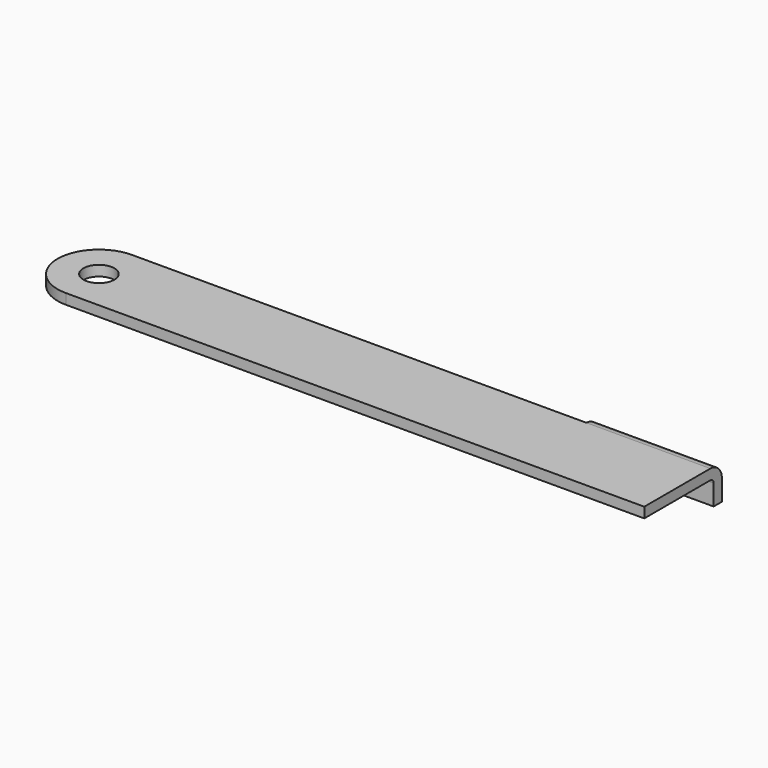
from build123d import *

# Parameters (mm, degrees)
F0_W     = 150
F0_H     = 20
F1_DEPTH = 2.5
F3_D     = 7.5
F4_R     = 9.99999
F5_W     = 2.5
F5_H     = 5
F6_DEPTH = 30


# Not quite as in the source:
# - a fillet or chamfer is up to 0.001 mm smaller than in the source, because OpenCascade refuses the exact size


with BuildPart() as f1:
    # F0 (on Top) → F1 (new body)
    with BuildSketch(Plane.XY):
        Rectangle(F0_W, F0_H)
    extrude(amount=F1_DEPTH)

    # F3 (through all)
    with Locations(Plane.XY.offset(2.5)):
        with Locations((-65, 0)):
            Hole(F3_D / 2)

    # F4 (radius 10 in the source; OpenCascade refuses exactly that, so slightly less here)
    f4_edges = [f1.edges().sort_by_distance(p)[0] for p in [
        (-75, -10, 1.25),
        (-75, 10, 1.25),
    ]]
    fillet(f4_edges, radius=F4_R)

    # F5 (on face) → F6 (join)
    with BuildSketch(Plane.YZ.offset(75)):
        with BuildLine():
            ThreePointArc((10, 0), (10.7071067812, -0.2928932188), (11, -1))
            Line((11, -1), (13.5, -1))
            ThreePointArc((13.5, -1), (12.4748737342, 1.4748737342), (10, 2.5))
            Line((10, 2.5), (10, 0))
        make_face()
        with Locations((12.25, -3.5)):
            Rectangle(F5_W, F5_H)
    extrude(amount=-F6_DEPTH)


solid = f1.part
